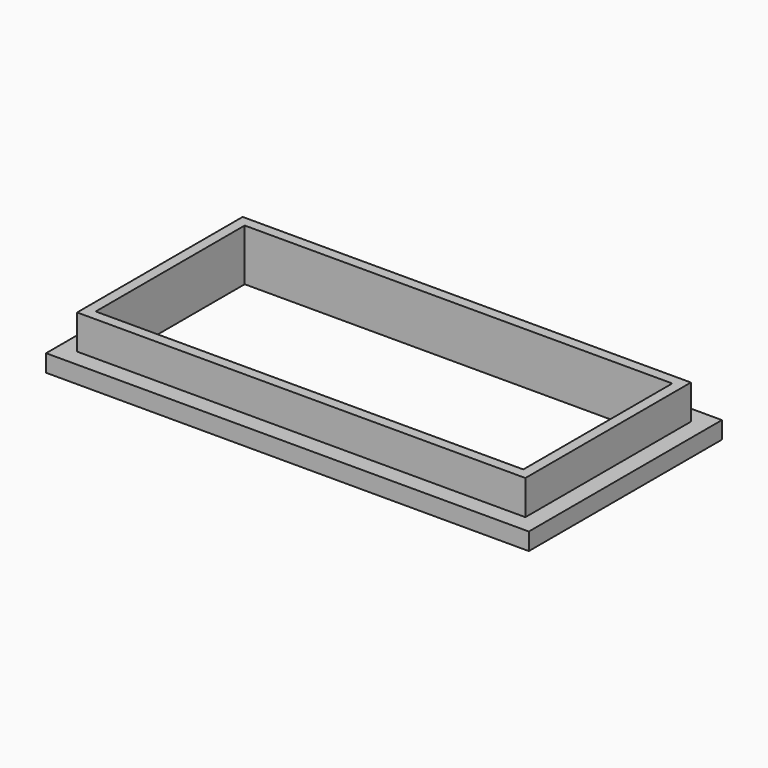
from build123d import *

# Parameters (mm, degrees)
F0_W     = 70
F0_H     = 35
F1_DEPTH = 2.5
F2_W     = 65
F2_H     = 30
F2_W_2   = 62
F2_H_2   = 27
F3_DEPTH = 5
F4_DEPTH = 2.5


# Not quite as in the source:
# - the program builds the solid bodies; features that only make, move or delete a surface that nothing else refers to are left out


with BuildPart() as f1:
    # F0 (on Top) → F1 (new body)
    with BuildSketch(Plane.XY):
        Rectangle(F0_W, F0_H)
    extrude(amount=F1_DEPTH)

    # F2 (on face) → F3 (join)
    with BuildSketch(Plane.XY.offset(2.5)):
        Rectangle(F2_W, F2_H)
        Rectangle(F2_W_2, F2_H_2, mode=Mode.SUBTRACT)
    extrude(amount=F3_DEPTH)

    # F4 (cut, through all): a face of the model
    f4_faces = [f1.faces().sort_by_distance(p)[0] for p in [
        (0, 0, 2.5),
    ]]
    extrude(f4_faces, amount=-F4_DEPTH, mode=Mode.SUBTRACT)


solid = f1.part
